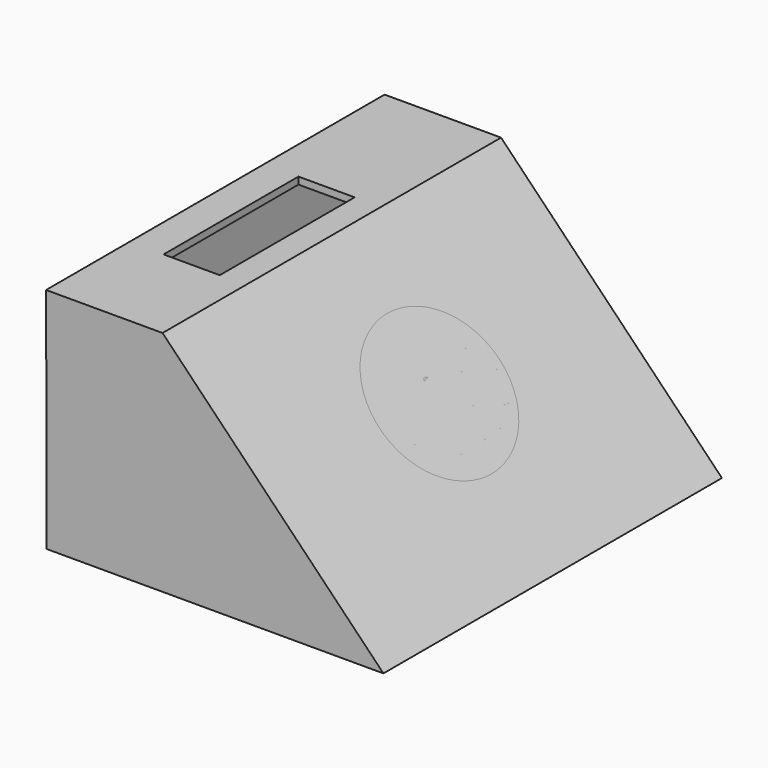
from build123d import *

# Parameters (mm, degrees)
F1_DEPTH = 152.4
F2_T     = -2.54
F3_R     = 26.9750626094
F5_DEPTH = 4.318
F4_W     = 20.2446002513
F4_H     = 60.7213377953
F6_DEPTH = 25.4


# Not quite as in the source:
# - a feature names something its author has since deleted; it is built from what else it names


with BuildPart() as f1:
    # F0 (on Front) → F1 (new body)
    with BuildSketch(Plane.XZ):
        Polygon((-59.7190245772, 46.653393656), (-59.4916790724, -35.4198999703), (61.7842264473, -35.4198999703), (-17.7672635764, 46.653393656), align=None)
    extrude(amount=F1_DEPTH)

    # F2
    f2_openings = [f1.faces().sort_by_distance(p)[0] for p in [
        (-15.567576, 0, -1.030813),
    ]]
    offset(amount=F2_T, openings=f2_openings)

    # F4 (on face) → F6 (cut)
    with BuildSketch(Plane.XY.offset(46.653393656)):
        with Locations((-37.3173421249, -84.4868421555)):
            Rectangle(F4_W, F4_H)
    extrude(amount=-F6_DEPTH, mode=Mode.SUBTRACT)


with BuildPart() as f5:
    # F3 (on face) → F5 (new body)
    with BuildSketch(Plane(origin=(14.1545580436, 0, 13.7196417159), x_dir=(0, 1, 0), z_dir=(0.7180522473, 0, 0.6959892026))):
        with Locations((-74.5968669653, -7.9793436453)):
            Circle(F3_R)
        Polygon((-76.937161386, -2.6940456592), (-76.9103467464, -2.5446491782), (-76.7360180616, -2.3765773512), (-76.6287446022, -2.096457174), (-76.5080600977, -2.096457174), (-76.4007866383, -1.9844097551), (-76.2398764491, -1.9844097551), (-76.0253220797, -1.9844097551), (-75.8510008454, -2.0030839369), (-75.7035017014, -1.9844097551), (-75.5828171968, -2.0030839369), (-75.4084959626, -2.0777829923), (-75.3280371428, -2.1898308769), (-75.1134902239, -2.2271808702), (-75.0196203589, -2.4139273446), (-74.8318955302, -2.581997076), (-75.1805379987, -2.4699498899), (-75.2878114581, -2.4699498899), (-75.4755437374, -2.3952506017), (-75.6364539266, -2.3952506017), (-75.7705494761, -2.3765773512), (-76.07896626, -2.3579027038), (-76.1460065842, -2.4699498899), (-76.3069242239, -2.581997076), (-76.4141976833, -2.8247681912), (-76.7092034221, -2.8060935438), (-76.8298879266, -2.8247681912), align=None, mode=Mode.SUBTRACT)
        with BuildLine():
            add(Edge.make_bspline(
                [(-73.7227074314, -1.1341697216), (-73.7176566552, -1.1319269484), (-73.7365462125, -1.127884318), (-73.7668424845, -1.1252524959)],
                knots=[0.0171389283, 0.0171389283, 0.0171389283, 0.0171389283, 0.1852596656, 0.1852596656, 0.1852596656, 0.1852596656], degree=3))
            add(Edge.make_bspline(
                [(-73.7250118097, -1.1347961173), (-73.7239860284, -1.1346082917), (-73.7232223286, -1.1343983593), (-73.7227074314, -1.1341697216)],
                knots=[0, 0, 0, 0, 0.0171389283, 0.0171389283, 0.0171389283, 0.0171389283], degree=3))
            add(Edge.make_bspline(
                [(-73.9545275863, -1.1243682694), (-73.9548856484, -1.1246478129), (-73.9510749235, -1.1298427137), (-73.7506281888, -1.1394866026), (-73.7250118097, -1.1347961173)],
                knots=[0.5462143148, 0.5462143148, 0.5462143148, 0.5462143148, 0.5719972033, 1, 1, 1, 1], degree=3))
            add(Edge.make_bspline(
                [(-73.7668424845, -1.1252524959), (-73.8318884771, -1.1196019828), (-73.9495147977, -1.1204547232), (-73.9545275863, -1.1243682694)],
                knots=[0.1852596656, 0.1852596656, 0.1852596656, 0.1852596656, 0.5462143148, 0.5462143148, 0.5462143148, 0.5462143148], degree=3))
        make_face(mode=Mode.SUBTRACT)
    extrude(amount=-F5_DEPTH)


solid = Compound([f1.part, f5.part])
